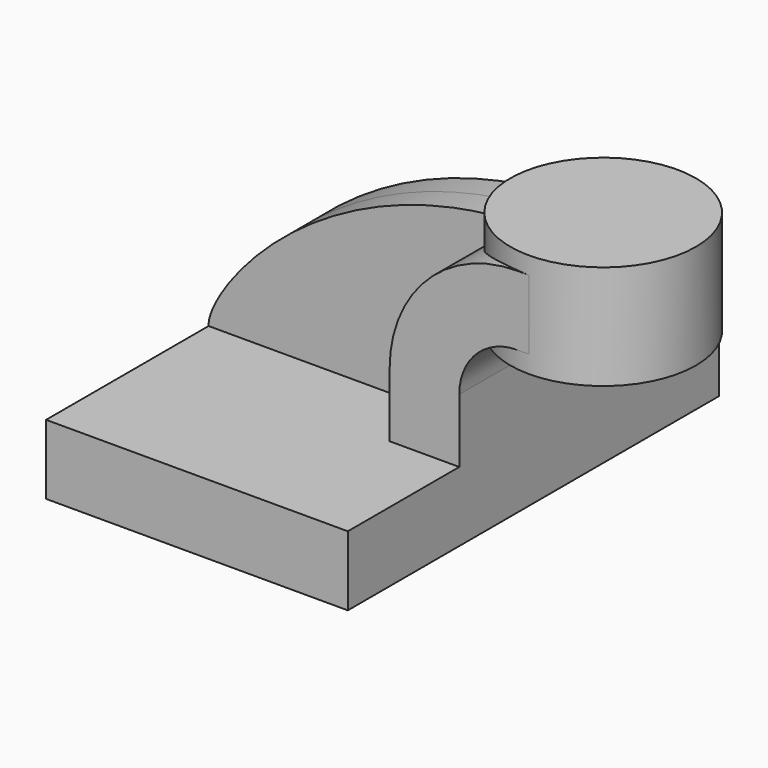
from build123d import *

# Parameters (mm, degrees)
F1_DEPTH = 63.5
F2_DEPTH = 25.4
F3_DEPTH = 7.9375
F0_W     = 25.4
F0_H     = 4.7498
F0_H_2   = 19.05
F0_H_3   = 4.7752


# Not quite as in the source:
# - a feature names something its author has since deleted; it is built from what else it names


with BuildPart() as f1:
    # F0 (on Front) → F1 (new body, symmetric)
    with BuildSketch(Plane.XZ):
        Polygon((-41.275, -9.525), (41.275, -9.525), (41.275, 9.525), (22.225, 9.525), (-41.275, 9.525), align=None)
    extrude(amount=F1_DEPTH, both=True)

    # F0 (on Front) → F2 (join, symmetric)
    with BuildSketch(Plane.XZ):
        with BuildLine():
            Line((22.225, 9.525), (41.275, 9.525))
            Line((41.275, 9.525), (41.275, 27.0002))
            ThreePointArc((41.275, 27.0002), (45.9246798487, 38.2255201513), (57.15, 42.8752))
            Line((57.15, 42.8752), (60.325, 42.8752))
            Line((60.325, 42.8752), (60.325, 61.9252))
            Line((60.325, 61.9252), (57.15, 61.9252))
            ThreePointArc((57.15, 61.9252), (32.4542956671, 51.6959043329), (22.225, 27.0002))
            Line((22.225, 27.0002), (22.225, 9.525))
        make_face()
    extrude(amount=F2_DEPTH, both=True)

    # F0 (on Front) → F3 (join, symmetric)
    with BuildSketch(Plane.XZ):
        with BuildLine():
            add(Edge.make_bspline(
                [(-41.275, 9.525), (-41.7312111626, 19.5100846971), (-7.2445928525, 66.0155981062), (57.15, 61.9252)],
                knots=[0, 0, 0, 0, 111.5045361635, 111.5045361635, 111.5045361635, 111.5045361635], degree=3))
            Line((-41.275, 9.525), (22.225, 9.525))
            Line((22.225, 9.525), (22.225, 27.0002))
            ThreePointArc((22.225, 27.0002), (32.4542956671, 51.6959043329), (57.15, 61.9252))
        make_face()
    extrude(amount=F3_DEPTH, both=True)

    # F0 (on Front) → F4 (revolve)
    with BuildSketch(Plane.XZ):
        with Locations((73.025, 64.3001)):
            Rectangle(F0_W, F0_H)
        with Locations((73.025, 52.4002)):
            Rectangle(F0_W, F0_H_2)
        with Locations((73.025, 40.4876)):
            Rectangle(F0_W, F0_H_3)
    revolve(axis=Axis((60.325, 0, 52.3875), (0, 0, 1)))


solid = f1.part
